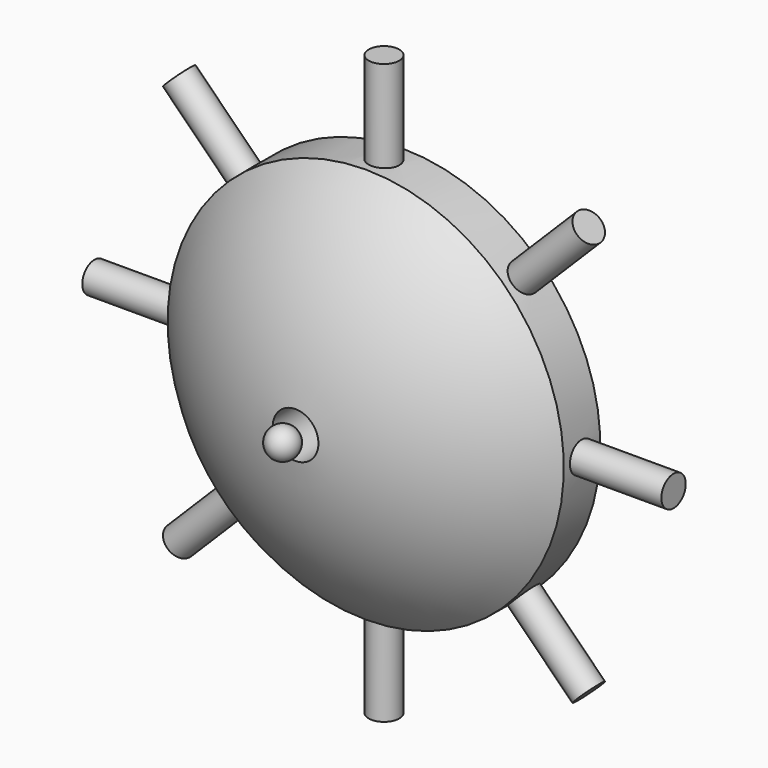
from build123d import *

# Parameters (mm, degrees)
F0_W     = 15
F0_H     = 65
F6_W     = 5
F6_H     = 30
F6_H_2   = 1.7657750845
F8_COUNT = 8
F10_D    = 15


with BuildPart() as f1:
    # F0 (on Right) → F1 (revolve)
    with BuildSketch(Plane.YZ):
        with Locations((-104.7048869729, 32.5)):
            Rectangle(F0_W, F0_H)
    revolve(axis=Axis((0, -59.3888796866, 0), (0, 1, 0)))

    # F2 (on Right) → F3 (revolve)
    with BuildSketch(Plane.YZ):
        with BuildLine():
            ThreePointArc((-141.2963948166, 0), (-133.6917758296, -35.6065858677), (-112.2048869729, -65))
            Line((-112.2048869729, -65), (-112.2048869729, 0))
            Line((-112.2048869729, 0), (-141.2963948166, 0))
        make_face()
    revolve(axis=Axis((0, -59.3888796866, 0), (0, 1, 0)))

    # F6 (on Right) → F7 (revolve)
    with BuildSketch(Plane.YZ):
        with Locations((-102.2048869729, 80)):
            Rectangle(F6_W, F6_H)
        with Locations((-102.2048869729, 64.1171124578)):
            Rectangle(F6_W, F6_H_2)
    revolve(axis=Axis((0, -104.7048869729, 87.7374348044), (0, 0, 1)))

    # F8: F1 ×8 about axis
    f8_axis = Axis((0, -59.3888796866, 0), (0, 1, 0))


with BuildPart() as f5:
    # F4 (on Right) → F5 (revolve)
    with BuildSketch(Plane.YZ):
        with BuildLine():
            Line((-151.2963948166, 0), (-141.2963948166, 0))
            ThreePointArc((-141.2963948166, 0), (-146.2963948166, 5), (-151.2963948166, 0))
        make_face()
    revolve(axis=Axis((0, -59.3888796866, 0), (0, 1, 0)))


with BuildPart() as f1_1:
    add(f1.part)
    for i in range(1, F8_COUNT):
        add(f1.part.rotate(f8_axis, i * 360 / F8_COUNT))

    # F10 (through all)
    with Locations(Plane(origin=(0, -97.2048869729, 0), x_dir=(-1, 0, 0), z_dir=(0, 1, 0))):
        with Locations((0, 0)):
            Hole(F10_D / 2)


solid = Compound([f5.part, f1_1.part])
